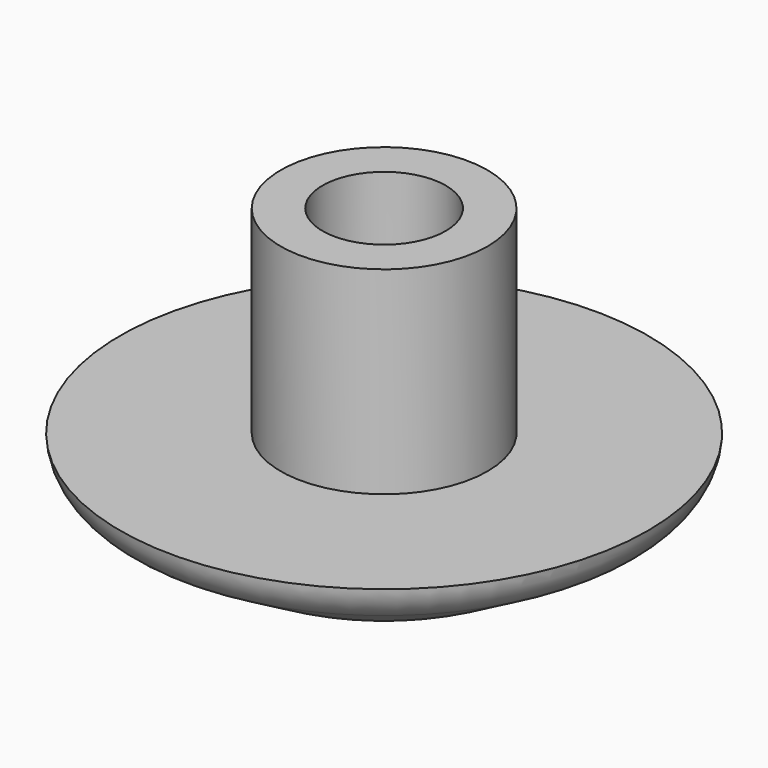
from build123d import *

# Parameters (mm, degrees)
F0_R     = 6
F1_DEPTH = 2
F2_SIZE2 = 2.5980762114
F2_SIZE  = 1.5
F4_R     = 2.35
F4_R_2   = 1.4
F5_DEPTH = 4.5
F6_R     = 1.2


# Not quite as in the source:
# - a fillet or chamfer that OpenCascade refuses, or shapes differently, is made with other operations: its cross-section is extruded or revolved along the edge and cut away or added


with BuildPart() as f1:
    # F0 (on Top) → F1 (new body)
    with BuildSketch(Plane.XY):
        Circle(F0_R)
    extrude(amount=F1_DEPTH)

    # F2
    f2_edges = [f1.edges().sort_by_distance(p)[0] for p in [
        (-6, 0, 0),
    ]]
    f2_side = f1.faces().sort_by_distance((-6, 0, 1))[0]
    chamfer(f2_edges, length=F2_SIZE, length2=F2_SIZE2, reference=f2_side)

    # F3: fillet of radius 1 on 2 edges, made by hand

    # F3_s1 → F3_t2 (revolve, cut)
    with BuildSketch(Plane.XZ):
        with BuildLine():
            ThreePointArc((3.6339745962, 0.1339745962), (3.3927936413, 0.0340741737), (3.1339745962, 0))
            Line((3.1339745962, 0), (3.4019237886, 0))
            Line((3.4019237886, 0), (3.6339745962, 0.1339745962))
        make_face()
    revolve(axis=Axis((0, 0, 0), (0, 0, 1)), mode=Mode.SUBTRACT)

    # F3_s3 → F3_t4 (revolve, cut)
    with BuildSketch(Plane.XZ):
        with BuildLine():
            ThreePointArc((6, 2), (5.8486778537, 1.5452494356), (5.5031382462, 1.2131367327))
            Line((5.5031382462, 1.2131367327), (6, 1.5))
            Line((6, 1.5), (6, 2))
        make_face()
    revolve(axis=Axis((0, 0, 1.5), (0, 0, 1)), mode=Mode.SUBTRACT)

    # F4 (on face) → F5 (join)
    with BuildSketch(Plane.XY.offset(2)):
        Circle(F4_R)
        Circle(F4_R_2, mode=Mode.SUBTRACT)
    extrude(amount=F5_DEPTH)

    # F6
    f6_edges = [f1.edges().sort_by_distance(p)[0] for p in [
        (-1.4, 0, 2),
    ]]
    fillet(f6_edges, radius=F6_R)


solid = f1.part
